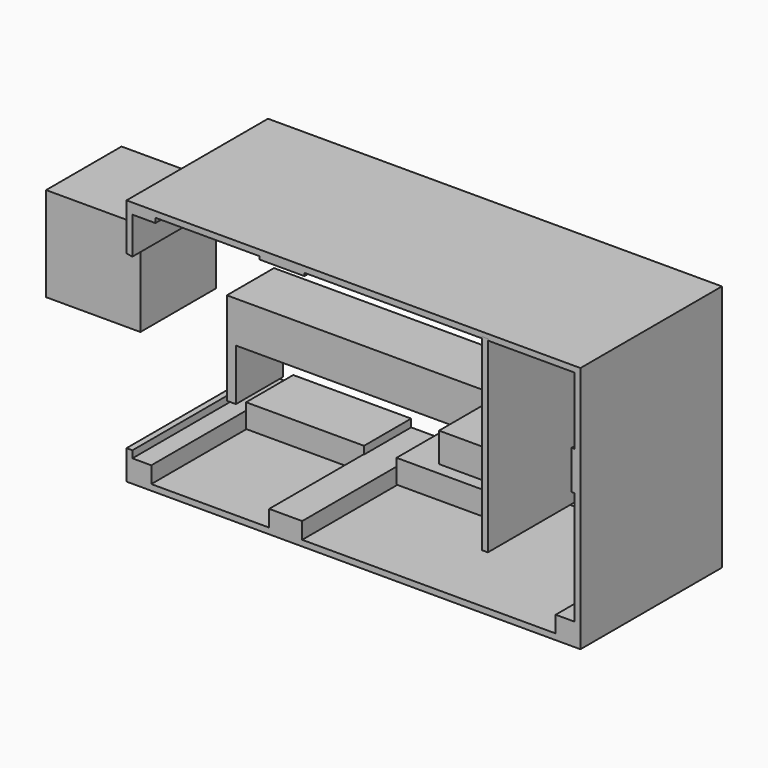
from build123d import *

# Parameters (mm, degrees)
F6_DEPTH  = 76.2
F5_W      = 2.54
F5_H      = 81.026
F1_W      = 139.7
F1_H      = 12.7
F7_DEPTH  = 25.4
F3_W      = 50.8
F3_H      = 10.16
F4_W      = 3.9116963744
F4_H      = 17.78
F4_W_2    = 123.0883036256
F4_H_2    = 22.2250012395
F2_W      = 38.1
F2_H      = 12.7
F8_DEPTH  = 50.8
F9_W      = 40.64
F9_H      = 40.64
F10_DEPTH = 40.64


with BuildPart() as f6:
    # F0 (on Front) → F6 (new body)
    with BuildSketch(Plane.XZ):
        Polygon((-74.6464829862, 55.9084560133), (-74.6464829862, 57.9404560133), (-29.7320684276, 57.9404560133), (-29.7320684276, 56.6704560133), (-10.4280684276, 56.6704560133), (-10.4280684276, 57.9404560133), (105.9475170138, 57.9404560133), (105.9475170138, 28.9844560133), (104.6775170138, 28.9844560133), (104.6775170138, 12.2204560133), (105.9475170138, 12.2204560133), (105.9475170138, -36.5475439867), (97.8195170138, -36.5475439867), (97.8195170138, -43.6595439867), (-11.4004829862, -43.6595439867), (-11.4004829862, -36.5475439867), (-25.6244829862, -36.5475439867), (-25.6244829862, -43.6595439867), (-76.4244829862, -43.6595439867), (-76.4244829862, -36.5475439867), (-84.5524829862, -36.5475439867), (-84.5524829862, -33.4995439867), (-87.0924829862, -33.4995439867), (-87.0924829862, -46.1995439867), (108.4875170138, -46.1995439867), (108.4875170138, -43.6595439867), (108.4875170138, 60.4804560133), (-87.0924829862, 60.4804560133), (-87.0924829862, 40.320412819), (-84.5524829862, 39.9525031491), (-84.5524829862, 55.9084560133), align=None)
    extrude(amount=F6_DEPTH)

    # F3 (on face) → F7, piece 2 (join)
    with BuildSketch(Plane.XZ):
        with Locations((-50.8139037251, -38.283083154)):
            Rectangle(F3_W, F3_H)
    extrude(amount=F7_DEPTH)


with BuildPart() as f6b:
    # F5 (on Front) → F6, piece 2 (new body)
    with BuildSketch(Plane.XZ):
        with Locations((67.3280618, 18.1041830366)):
            Rectangle(F5_W, F5_H)
    extrude(amount=F6_DEPTH)


with BuildPart() as f7:
    # F1 (on Front) → F7 (new body)
    with BuildSketch(Plane.XZ):
        with Locations((-4.0278486848, 49.8614082277)):
            Rectangle(F1_W, F1_H)
    extrude(amount=F7_DEPTH)


with BuildPart() as f7b:
    # F3 (on face) → F7, piece 3 (new body)
    with BuildSketch(Plane.XZ):
        with Locations((14.0117149144, -38.283083154)):
            Rectangle(F3_W, F3_H)
    extrude(amount=F7_DEPTH)


with BuildPart() as f7c:
    # F4 (on Front) → F7, piece 4 (new body)
    with BuildSketch(Plane.XZ):
        with Locations((-82.5479365885, -4.2277628699)):
            Rectangle(F4_W, F4_H)
        with Locations((-19.0479365885, -4.2277628699)):
            Rectangle(F4_W_2, F4_H)
        with Locations((-82.5479365885, -24.2302634896)):
            Rectangle(F4_W, F4_H_2)
    extrude(amount=F7_DEPTH)


with BuildPart() as f8:
    # F2 (on Front) → F8 (new body)
    with BuildSketch(Plane.XZ):
        with Locations((46.296966958, -6.35)):
            Rectangle(F2_W, F2_H)
    extrude(amount=F8_DEPTH)


with BuildPart() as f10:
    # F9 (on Front) → F10 (new body)
    with BuildSketch(Plane.XZ):
        with Locations((-129.8780011606, 9.0961520222)):
            Rectangle(F9_W, F9_H)
    extrude(amount=F10_DEPTH)


solid = Compound([f6.part, f6b.part, f7.part, f7b.part, f7c.part, f8.part, f10.part])
